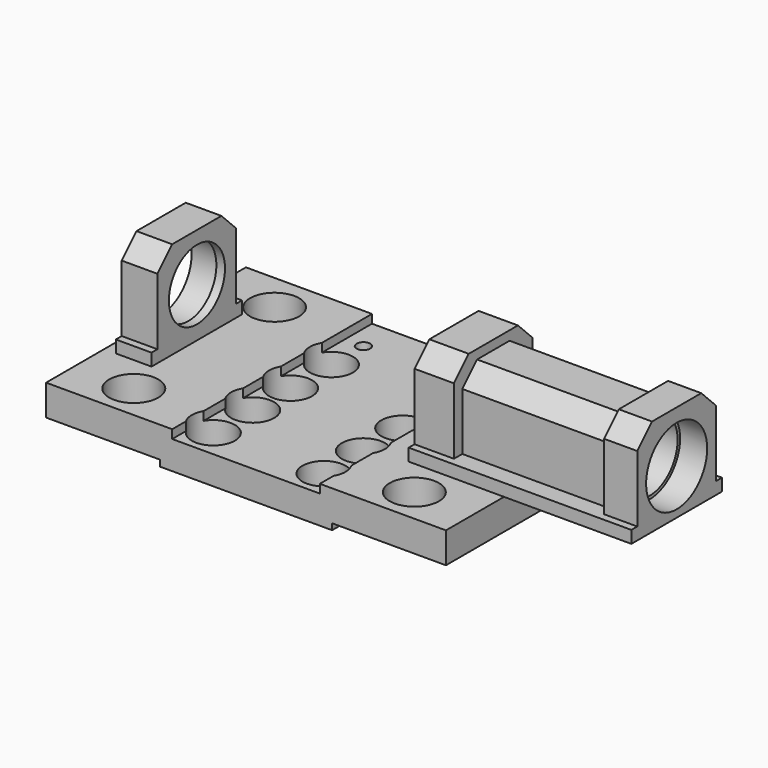
from build123d import *

# Parameters (mm, degrees)
F1_DEPTH  = 203
F4_DEPTH  = 29
F5_SIZE   = 15
F6_R      = 28.5
F7_DEPTH  = 7
F8_R      = 31
F9_DEPTH  = 22
F11_D     = 9
F11_DEPTH = 22
F11_TIP   = 2.7038727856
F12_D     = 40
F14_D     = 35
F15_D     = 11
F18_R     = 31
F19_DEPTH = 32
F20_SIZE  = 15
F21_R     = 31
F22_DEPTH = 122
F23_SIZE  = 15
F24_R     = 31
F25_DEPTH = 27
F26_SIZE  = 15
F28_D     = 5.5
F28_DEPTH = 10
F28_TIP   = 1.6523667023
F29_R     = 31
F30_DEPTH = 181
F31_R     = 31
F32_DEPTH = 5
F33_DEPTH = 27
F34_R     = 28.5
F35_DEPTH = 154
F36_R     = 31
F36_R_2   = 28.5
F37_DEPTH = 22


with BuildPart() as f1:
    # F0 (on Front) → F1 (new body)
    with BuildSketch(Plane.XZ):
        Polygon((0, 25), (0, 0), (92.5, 0), (92.5, -5), (232.5, -5), (232.5, 0), (325, 0), (325, 25), (222.5, 25), (222.5, 18), (102.5, 18), (102.5, 25), align=None)
    extrude(amount=-F1_DEPTH)

    # F3 (on offset) → F4 (join)
    with BuildSketch(Plane.YZ.offset(38.5)):
        Polygon((59, 25), (151, 25), (151, 35), (145, 35), (145, 104), (65, 104), (65, 35), (59, 35), align=None)
    extrude(amount=-F4_DEPTH)

    # F5
    f5_edges = [f1.edges().sort_by_distance(p)[0] for p in [
        (24, 65, 104),
        (24, 145, 104),
    ]]
    chamfer(f5_edges, length=F5_SIZE)

    # F6 (on face) → F7 (cut)
    with BuildSketch(Plane.YZ.offset(38.5)):
        with Locations((105.1451787353, 65)):
            Circle(F6_R)
    extrude(amount=-F7_DEPTH, mode=Mode.SUBTRACT)

    # F8 (on face) → F9 (cut)
    with BuildSketch(Plane(origin=(9.5, 0, 0), x_dir=(0, -1, 0), z_dir=(-1, 0, 0))):
        with Locations((-105, 65)):
            Circle(F8_R)
    extrude(amount=-F9_DEPTH, mode=Mode.SUBTRACT)

    # F11
    with Locations(Plane(origin=(0, 0, 0), x_dir=(1, 0, 0), z_dir=(0, 0, -1))):
        with Locations((12.5, -182), (12.5, -130), (12.5, -73), (12.5, -21), (84.5, -73), (84.5, -130), (84.5, -182), (240.5, -182), (312.5, -182), (240.5, -130), (312.5, -130), (240.5, -73), (312.5, -73), (240.5, -21), (312.5, -21), (84.5, -21)):
            Hole(F11_D / 2, depth=F11_DEPTH)
            with Locations((0, 0, -(F11_DEPTH + F11_TIP / 2))):  # 118° drill point
                Cone(0, F11_D / 2, F11_TIP, mode=Mode.SUBTRACT)

    # F12 (through all)
    with Locations(Plane(origin=(0, 0, 0), x_dir=(1, 0, 0), z_dir=(0, 0, -1))):
        with Locations((48.5, -28.5), (48.5, -171.5), (276.5, -28.5), (276.5, -171.5)):
            Hole(F12_D / 2)

    # F14 (through all)
    with Locations(Plane(origin=(0, 0, -5), x_dir=(1, 0, 0), z_dir=(0, 0, -1))):
        with Locations((117.5, -23), (117.5, -63), (117.5, -143), (207.5, -143), (207.5, -103), (117.5, -101.5), (207.5, -63), (207.5, -23)):
            Hole(F14_D / 2)

    # F15 (through all)
    with Locations(Plane(origin=(0, 0, -5), x_dir=(1, 0, 0), z_dir=(0, 0, -1))):
        with Locations((117.5, -175.5), (207.5, -175.5)):
            Hole(F15_D / 2)

    # F18 (on offset) → F19 (join)
    with BuildSketch(Plane.YZ.offset(247.5)):
        Polygon((59, 25), (151, 25), (151, 35), (145, 35), (145, 104), (65, 104), (65, 35), (59, 35), align=None)
        with Locations((105.1451787353, 65)):
            Circle(F18_R, mode=Mode.SUBTRACT)
    extrude(amount=F19_DEPTH)

    # F20
    f20_edges = [f1.edges().sort_by_distance(p)[0] for p in [
        (263.5, 65, 104),
        (263.5, 145, 104),
    ]]
    chamfer(f20_edges, length=F20_SIZE)

    # F21 (on face) → F22 (join)
    with BuildSketch(Plane.YZ.offset(279.5)):
        Polygon((151, 35), (145, 35), (136.5, 35), (136.5, 96.5), (73.5, 96.5), (73.5, 35), (65, 35), (59, 35), (59, 25), (151, 25), align=None)
        with Locations((105.1451787353, 65)):
            Circle(F21_R, mode=Mode.SUBTRACT)
    extrude(amount=F22_DEPTH)

    # F23
    f23_edges = [f1.edges().sort_by_distance(p)[0] for p in [
        (340.5, 73.5, 96.5),
        (340.5, 136.5, 96.5),
    ]]
    chamfer(f23_edges, length=F23_SIZE)

    # F24 (on face) → F25 (join)
    with BuildSketch(Plane.YZ.offset(401.5)):
        Polygon((65, 104), (65, 35), (73.5, 35), (73.5, 81.5), (88.5, 96.5), (121.5, 96.5), (136.5, 81.5), (136.5, 35), (145, 35), (145, 104), align=None)
        Polygon((59, 35), (59, 25), (151, 25), (151, 35), (145, 35), (136.5, 35), (136.5, 81.5), (121.5, 96.5), (88.5, 96.5), (73.5, 81.5), (73.5, 35), (65, 35), align=None)
        with Locations((105.1451787353, 65)):
            Circle(F24_R, mode=Mode.SUBTRACT)
    extrude(amount=F25_DEPTH)

    # F26
    f26_edges = [f1.edges().sort_by_distance(p)[0] for p in [
        (415, 65, 104),
        (415, 145, 104),
    ]]
    chamfer(f26_edges, length=F26_SIZE)

    # F28
    with Locations(Plane(origin=(9.5, 0, 0), x_dir=(0, -1, 0), z_dir=(-1, 0, 0))):
        with Locations((-130, 89.5), (-80, 89.5), (-130, 39.5), (-80, 39.5)):
            Hole(F28_D / 2, depth=F28_DEPTH)
            with Locations((0, 0, -(F28_DEPTH + F28_TIP / 2))):  # 118° drill point
                Cone(0, F28_D / 2, F28_TIP, mode=Mode.SUBTRACT)

    # F29 (on face) → F30 (join)
    with BuildSketch(Plane.YZ.offset(428.5)):
        with Locations((105.1451787353, 65)):
            Circle(F29_R)
    extrude(amount=-F30_DEPTH)

    # F31 (on face) → F32 (join)
    with BuildSketch(Plane(origin=(247.5, 0, 0), x_dir=(0, -1, 0), z_dir=(-1, 0, 0))):
        with Locations((-105, 62)):
            Circle(F31_R)
    extrude(amount=-F32_DEPTH)

    # F31 (on face) → F33 (cut)
    with BuildSketch(Plane(origin=(247.5, 0, 0), x_dir=(0, -1, 0), z_dir=(-1, 0, 0))):
        with Locations((-105, 62)):
            Circle(F31_R)
    extrude(amount=-F33_DEPTH, mode=Mode.SUBTRACT)

    # F34 (on face) → F35 (cut)
    with BuildSketch(Plane.YZ.offset(428.5)):
        with Locations((105, 62)):
            Circle(F34_R)
    extrude(amount=-F35_DEPTH, mode=Mode.SUBTRACT)

    # F36 (on face) → F37 (cut)
    with BuildSketch(Plane.YZ.offset(428.5)):
        with Locations((105, 62)):
            Circle(F36_R)
        with Locations((105, 62)):
            Circle(F36_R_2, mode=Mode.SUBTRACT)
    extrude(amount=-F37_DEPTH, mode=Mode.SUBTRACT)


solid = f1.part
